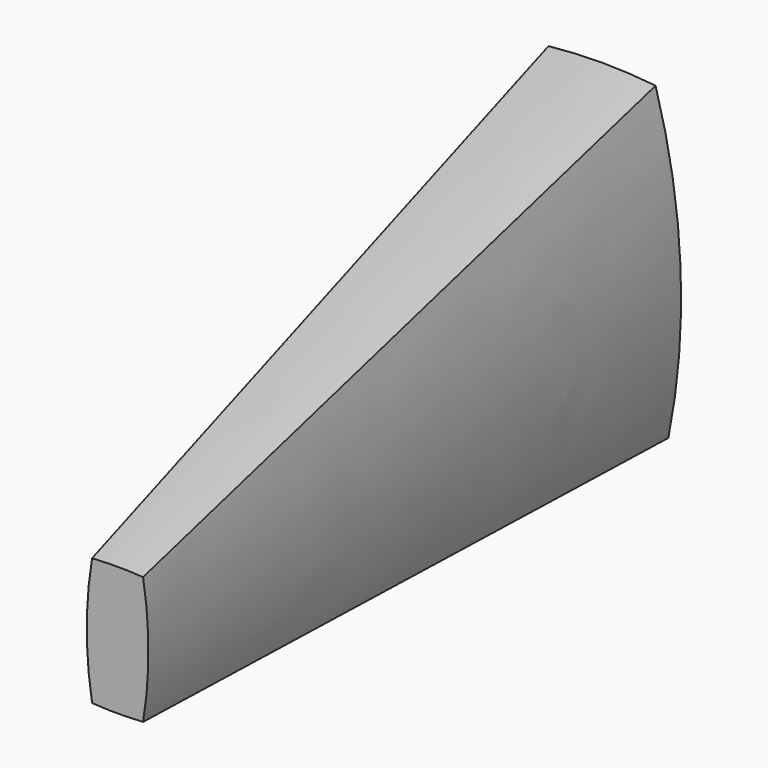
from build123d import *


with BuildPart() as f3:
    # F0 (on Front) → F3 section 0
    with BuildSketch(Plane.XZ):
        with BuildLine():
            ThreePointArc((21, 60), (0, 61.1055556331), (-21, 60))
            ThreePointArc((-21, 60), (-30.8133090839, 0.3047212118), (-26, -60))
            ThreePointArc((-26, -60), (0, -61.69720123), (26, -60))
            ThreePointArc((26, -60), (30.8133090839, 0.3047212118), (21, 60))
        make_face()
    # F2 (on offset) → F3 section 1
    with BuildSketch(Plane.XZ.offset(300)):
        with BuildLine():
            ThreePointArc((60.0354610384, 25), (50.0354610384, 25.333704529), (40.0354610384, 25))
            ThreePointArc((40.0354610384, 25), (37.9374556158, 0), (40.0354610384, -25))
            ThreePointArc((40.0354610384, -25), (50.0354610384, -25.333704529), (60.0354610384, -25))
            ThreePointArc((60.0354610384, -25), (62.1334664609, 0), (60.0354610384, 25))
        make_face()
    loft()


solid = f3.part
